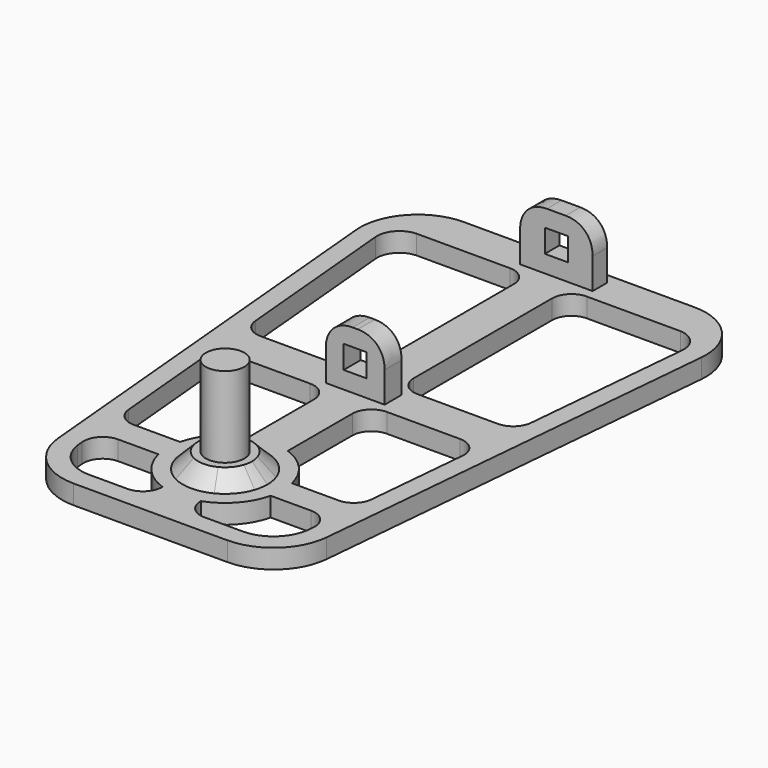
from build123d import *

# Parameters (mm, degrees)
F1_DEPTH    = 6.35
F2_DEPTH    = 25.4
F3_T1_DEPTH = 51.4821597159
F3_T3_DEPTH = 50.4775569558
F5_DEPTH    = 92.5147765378
F0_R        = 6.35
F6_DEPTH    = 11.43
F7_SIZE     = 5.07999
F8_DEPTH    = 38.1


# Not quite as in the source:
# - a fillet or chamfer that OpenCascade refuses, or shapes differently, is made with other operations: its cross-section is extruded or revolved along the edge and cut away or added
# - a fillet or chamfer is up to 0.001 mm smaller than in the source, because OpenCascade refuses the exact size


with BuildPart() as f1:
    # F0 (on Top) → F1 (new body)
    with BuildSketch(Plane.XY):
        with BuildLine():
            Line((38.1, 88.9586370111), (0, 88.9586370111))
            Line((0, 88.9586370111), (-38.1, 88.9586370111))
            ThreePointArc((-38.1, 88.9586370111), (-52.1700244652, 82.7514136403), (-57.0709376771, 68.1748481972))
            Line((-57.0709376771, 68.1748481972), (-44.3709376771, -70.7872367892))
            ThreePointArc((-44.3709376771, -70.7872367892), (-38.2427766292, -83.1234724406), (-25.4, -88.1034479753))
            Line((-25.4, -88.1034479753), (0, -88.1034479753))
            Line((0, -88.1034479753), (25.4, -88.1034479753))
            ThreePointArc((25.4, -88.1034479753), (38.2427766292, -83.1234724406), (44.3709376771, -70.7872367892))
            Line((44.3709376771, -70.7872367892), (57.0709376771, 68.1748481972))
            ThreePointArc((57.0709376771, 68.1748481972), (52.1700244652, 82.7514136403), (38.1, 88.9586370111))
        make_face()
        with BuildLine():
            Line((-12.7, -81.7534479753), (-25.4, -81.7534479753))
            ThreePointArc((-25.4, -81.7534479753), (-33.7498286884, -78.6277029444), (-37.9944737374, -70.7872367892))
            Line((-37.9944737374, -70.7872367892), (-38.1945348322, -68.5981890052))
            ThreePointArc((-38.1945348322, -68.5981890052), (-36.5608970949, -63.7393338575), (-31.8708889399, -61.6702594006))
            Line((-31.8708889399, -61.6702594006), (-18.54215425, -61.6702594006))
            ThreePointArc((-18.54215425, -61.6702594006), (-19.0498410445, -57.2231112436), (-18.5058372648, -52.7802594006))
            Line((-18.5058372648, -52.7802594006), (-33.8440386665, -52.7802594006))
            ThreePointArc((-33.8440386665, -52.7802594006), (-38.1249642095, -51.1202675557), (-40.1676845588, -47.0081890052))
            Line((-40.1676845588, -47.0081890052), (-43.2503548745, -13.2779296046))
            ThreePointArc((-43.2503548745, -13.2779296046), (-41.6167171372, -8.4190744569), (-36.9267089821, -6.35))
            Line((-36.9267089821, -6.35), (-12.7, -6.35))
            ThreePointArc((-12.7, -6.35), (-8.2098719395, -8.2098719395), (-6.35, -12.7))
            Line((-6.35, -12.7), (-6.35, -39.3404204633))
            ThreePointArc((-6.35, -39.3404204633), (0, -38.2509327054), (6.35, -39.3404204633))
            Line((6.35, -39.3404204633), (6.35, -12.7))
            ThreePointArc((6.35, -12.7), (8.2098719395, -8.2098719395), (12.7, -6.35))
            Line((12.7, -6.35), (36.9267089821, -6.35))
            ThreePointArc((36.9267089821, -6.35), (41.6167171372, -8.4190744569), (43.2503548745, -13.2779296046))
            Line((43.2503548745, -13.2779296046), (40.1676845588, -47.0081890052))
            ThreePointArc((40.1676845588, -47.0081890052), (38.1249642095, -51.1202675557), (33.8440386665, -52.7802594006))
            Line((33.8440386665, -52.7802594006), (18.5058372648, -52.7802594006))
            ThreePointArc((18.5058372648, -52.7802594006), (18.9134700663, -55.0242794484), (19.05, -57.3009327054))
            ThreePointArc((19.05, -57.3009327054), (18.9226126428, -59.5003032446), (18.54215425, -61.6702594006))
            Line((18.54215425, -61.6702594006), (31.8708889399, -61.6702594006))
            ThreePointArc((31.8708889399, -61.6702594006), (36.5608970949, -63.7393338575), (38.1945348322, -68.5981890052))
            Line((38.1945348322, -68.5981890052), (37.9944737374, -70.7872367892))
            ThreePointArc((37.9944737374, -70.7872367892), (33.7498286884, -78.6277029444), (25.4, -81.7534479753))
            Line((25.4, -81.7534479753), (12.7, -81.7534479753))
            ThreePointArc((12.7, -81.7534479753), (8.2098719395, -79.8935760359), (6.35, -75.4034479753))
            Line((6.35, -75.4034479753), (6.35, -75.2614449475))
            ThreePointArc((6.35, -75.2614449475), (0, -76.3509327054), (-6.35, -75.2614449475))
            Line((-6.35, -75.2614449475), (-6.35, -75.4034479753))
            ThreePointArc((-6.35, -75.4034479753), (-8.2098719395, -79.8935760359), (-12.7, -81.7534479753))
        make_face(mode=Mode.SUBTRACT)
        Polygon((-9.7281606868, 3.4770201892), (0, 3.4770201892), (9.7281606868, 3.4770201892), (9.7281606868, -3.5551395267), (0, -3.5551395267), (-9.7281606868, -3.5551395267), align=None, mode=Mode.SUBTRACT)
        with BuildLine():
            Line((-45.571707494, 12.1220703954), (-50.6944737374, 68.1748481972))
            ThreePointArc((-50.6944737374, 68.1748481972), (-48.902422759, 73.7198976746), (-43.6570607126, 76.2586370111))
            Line((-43.6570607126, 76.2586370111), (-12.7, 76.2586370111))
            ThreePointArc((-12.7, 76.2586370111), (-8.2098719395, 74.3987650716), (-6.35, 69.9086370111))
            Line((-6.35, 69.9086370111), (-6.35, 12.7))
            ThreePointArc((-6.35, 12.7), (-8.2098719395, 8.2098719395), (-12.7, 6.35))
            Line((-12.7, 6.35), (-39.2480616016, 6.35))
            ThreePointArc((-39.2480616016, 6.35), (-43.5289871447, 8.0099918449), (-45.571707494, 12.1220703954))
        make_face(mode=Mode.SUBTRACT)
        with BuildLine():
            Line((6.35, 12.7), (6.35, 69.9086370111))
            ThreePointArc((6.35, 69.9086370111), (8.2098719395, 74.3987650716), (12.7, 76.2586370111))
            Line((12.7, 76.2586370111), (43.6570607126, 76.2586370111))
            ThreePointArc((43.6570607126, 76.2586370111), (48.902422759, 73.7198976746), (50.6944737374, 68.1748481972))
            Line((50.6944737374, 68.1748481972), (45.571707494, 12.1220703954))
            ThreePointArc((45.571707494, 12.1220703954), (43.5289871447, 8.0099918449), (39.2480616016, 6.35))
            Line((39.2480616016, 6.35), (12.7, 6.35))
            ThreePointArc((12.7, 6.35), (8.2098719395, 8.2098719395), (6.35, 12.7))
        make_face(mode=Mode.SUBTRACT)
        Polygon((-11.9884992018, 85.6025964022), (0, 85.6025964022), (11.9884992018, 85.6025964022), (11.9884992018, 79.5750394464), (0, 79.5750394464), (-11.9884992018, 79.5750394464), align=None, mode=Mode.SUBTRACT)
        with BuildLine():
            Line((-6.35, -69.7443405987), (-6.35, -75.2614449475))
            ThreePointArc((-6.35, -75.2614449475), (0, -76.3509327054), (6.35, -75.2614449475))
            Line((6.35, -75.2614449475), (6.35, -69.7443405987))
            ThreePointArc((6.35, -69.7443405987), (0, -71.2709327054), (-6.35, -69.7443405987))
        make_face()
        with BuildLine():
            Line((6.35, -69.7443405987), (6.35, -75.2614449475))
            ThreePointArc((6.35, -75.2614449475), (14.1804413522, -70.021686734), (18.54215425, -61.6702594006))
            Line((18.54215425, -61.6702594006), (13.2691327611, -61.6702594006))
            ThreePointArc((13.2691327611, -61.6702594006), (10.6077938033, -66.3913458218), (6.35, -69.7443405987))
        make_face()
        with BuildLine():
            Line((13.2691327611, -61.6702594006), (18.54215425, -61.6702594006))
            ThreePointArc((18.54215425, -61.6702594006), (18.9226126428, -59.5003032446), (19.05, -57.3009327054))
            ThreePointArc((19.05, -57.3009327054), (18.9134700663, -55.0242794484), (18.5058372648, -52.7802594006))
            Line((18.5058372648, -52.7802594006), (13.2183362369, -52.7802594006))
            ThreePointArc((13.2183362369, -52.7802594006), (13.7808029017, -55.0095638164), (13.97, -57.3009327054))
            ThreePointArc((13.97, -57.3009327054), (13.7936703722, -59.5135234186), (13.2691327611, -61.6702594006))
        make_face()
        with BuildLine():
            ThreePointArc((18.5058372648, -52.7802594006), (14.1283572718, -44.522356071), (6.35, -39.3404204633))
            Line((6.35, -39.3404204633), (6.35, -44.8575248121))
            ThreePointArc((6.35, -44.8575248121), (10.555679827, -48.1500571522), (13.2183362369, -52.7802594006))
            Line((13.2183362369, -52.7802594006), (18.5058372648, -52.7802594006))
        make_face()
        with BuildLine():
            ThreePointArc((-6.35, -39.3404204633), (-14.1283572718, -44.522356071), (-18.5058372648, -52.7802594006))
            Line((-18.5058372648, -52.7802594006), (-13.2183362369, -52.7802594006))
            ThreePointArc((-13.2183362369, -52.7802594006), (-10.555679827, -48.1500571522), (-6.35, -44.8575248121))
            Line((-6.35, -44.8575248121), (-6.35, -39.3404204633))
        make_face()
        with BuildLine():
            ThreePointArc((-18.54215425, -61.6702594006), (-14.1804413522, -70.021686734), (-6.35, -75.2614449475))
            Line((-6.35, -75.2614449475), (-6.35, -69.7443405987))
            ThreePointArc((-6.35, -69.7443405987), (-10.6077938033, -66.3913458218), (-13.2691327611, -61.6702594006))
            Line((-13.2691327611, -61.6702594006), (-18.54215425, -61.6702594006))
        make_face()
        with BuildLine():
            ThreePointArc((-18.5058372648, -52.7802594006), (-19.0498410445, -57.2231112436), (-18.54215425, -61.6702594006))
            Line((-18.54215425, -61.6702594006), (-13.2691327611, -61.6702594006))
            ThreePointArc((-13.2691327611, -61.6702594006), (-13.9697719552, -57.221110899), (-13.2183362369, -52.7802594006))
            Line((-13.2183362369, -52.7802594006), (-18.5058372648, -52.7802594006))
        make_face()
        with BuildLine():
            ThreePointArc((6.35, -39.3404204633), (0, -38.2509327054), (-6.35, -39.3404204633))
            Line((-6.35, -39.3404204633), (-6.35, -44.8575248121))
            ThreePointArc((-6.35, -44.8575248121), (0, -43.3309327054), (6.35, -44.8575248121))
            Line((6.35, -44.8575248121), (6.35, -39.3404204633))
        make_face()
    extrude(amount=F1_DEPTH)

    # F0 (on Top) → F2 (join)
    with BuildSketch(Plane.XY):
        Polygon((9.7281606868, 3.4770201892), (0, 3.4770201892), (-9.7281606868, 3.4770201892), (-9.7281606868, -3.5551395267), (0, -3.5551395267), (9.7281606868, -3.5551395267), align=None)
        Polygon((11.9884992018, 85.6025964022), (0, 85.6025964022), (-11.9884992018, 85.6025964022), (-11.9884992018, 79.5750394464), (0, 79.5750394464), (11.9884992018, 79.5750394464), align=None)
    extrude(amount=F2_DEPTH)

    # F3: fillet of radius 8.89 on 4 edges, made by hand

    # F3_s2 → F3_t1 (cut)
    with BuildSketch(Plane.XZ.offset(-25.7020201892)):
        with BuildLine():
            add(Edge.make_bspline(
                [(-9.7281606868, 16.51), (-9.7281606868, 25.4), (-0.8381606868, 25.4)],
                knots=[0, 0, 0, 1, 1, 1], degree=2, weights=[1, 0.8181818182, 1]))
            Line((-0.8381606868, 25.4), (-9.7281606868, 25.4))
            Line((-9.7281606868, 25.4), (-9.7281606868, 16.51))
        make_face()
        with BuildLine():
            add(Edge.make_bspline(
                [(9.7281606868, 16.51), (9.7281606868, 25.4), (0.8381606868, 25.4)],
                knots=[0, 0, 0, 1, 1, 1], degree=2, weights=[1, 0.8181818182, 1]))
            Line((0.8381606868, 25.4), (9.7281606868, 25.4))
            Line((9.7281606868, 25.4), (9.7281606868, 16.51))
        make_face()
    extrude(amount=F3_T1_DEPTH, mode=Mode.SUBTRACT)

    # F3_s4 → F3_t3 (cut)
    with BuildSketch(Plane.XZ.offset(-107.8275964022)):
        with BuildLine():
            add(Edge.make_bspline(
                [(11.9884992018, 16.51), (11.9884992018, 25.4), (3.0984992018, 25.4)],
                knots=[0, 0, 0, 1, 1, 1], degree=2, weights=[1, 0.8181818182, 1]))
            Line((3.0984992018, 25.4), (11.9884992018, 25.4))
            Line((11.9884992018, 25.4), (11.9884992018, 16.51))
        make_face()
        with BuildLine():
            add(Edge.make_bspline(
                [(-11.9884992018, 16.51), (-11.9884992018, 25.4), (-3.0984992018, 25.4)],
                knots=[0, 0, 0, 1, 1, 1], degree=2, weights=[1, 0.8181818182, 1]))
            Line((-3.0984992018, 25.4), (-11.9884992018, 25.4))
            Line((-11.9884992018, 25.4), (-11.9884992018, 16.51))
        make_face()
    extrude(amount=F3_T3_DEPTH, mode=Mode.SUBTRACT)

    # F4 (on face) → F5 (cut, through all)
    with BuildSketch(Plane.XZ.offset(3.5551395267)):
        Polygon((3.81, 19.685), (0, 19.685), (-3.81, 19.685), (-3.81, 15.875), (-3.81, 12.065), (0, 12.065), (3.81, 12.065), (3.81, 15.875), align=None)
    extrude(amount=-F5_DEPTH, mode=Mode.SUBTRACT)

    # F0 (on Top) → F6 (join)
    with BuildSketch(Plane.XY):
        with BuildLine():
            Line((-6.35, -61.6702594006), (-6.35, -69.7443405987))
            ThreePointArc((-6.35, -69.7443405987), (0, -71.2709327054), (6.35, -69.7443405987))
            Line((6.35, -69.7443405987), (6.35, -61.6702594006))
            Line((6.35, -61.6702594006), (13.2691327611, -61.6702594006))
            ThreePointArc((13.2691327611, -61.6702594006), (13.7936703722, -59.5135234186), (13.97, -57.3009327054))
            ThreePointArc((13.97, -57.3009327054), (13.7808029017, -55.0095638164), (13.2183362369, -52.7802594006))
            Line((13.2183362369, -52.7802594006), (6.35, -52.7802594006))
            Line((6.35, -52.7802594006), (6.35, -44.8575248121))
            ThreePointArc((6.35, -44.8575248121), (0, -43.3309327054), (-6.35, -44.8575248121))
            Line((-6.35, -44.8575248121), (-6.35, -52.7802594006))
            Line((-6.35, -52.7802594006), (-13.2183362369, -52.7802594006))
            ThreePointArc((-13.2183362369, -52.7802594006), (-13.9697719552, -57.221110899), (-13.2691327611, -61.6702594006))
            Line((-13.2691327611, -61.6702594006), (-6.35, -61.6702594006))
        make_face()
        with Locations((0, -57.3009327054)):
            Circle(F0_R, mode=Mode.SUBTRACT)
        with BuildLine():
            ThreePointArc((-6.35, -44.8575248121), (-10.555679827, -48.1500571522), (-13.2183362369, -52.7802594006))
            Line((-13.2183362369, -52.7802594006), (-6.35, -52.7802594006))
            Line((-6.35, -52.7802594006), (-6.35, -44.8575248121))
        make_face()
        with BuildLine():
            ThreePointArc((-13.2691327611, -61.6702594006), (-10.6077938033, -66.3913458218), (-6.35, -69.7443405987))
            Line((-6.35, -69.7443405987), (-6.35, -61.6702594006))
            Line((-6.35, -61.6702594006), (-13.2691327611, -61.6702594006))
        make_face()
        with BuildLine():
            ThreePointArc((13.2183362369, -52.7802594006), (10.555679827, -48.1500571522), (6.35, -44.8575248121))
            Line((6.35, -44.8575248121), (6.35, -52.7802594006))
            Line((6.35, -52.7802594006), (13.2183362369, -52.7802594006))
        make_face()
        with BuildLine():
            Line((6.35, -61.6702594006), (6.35, -69.7443405987))
            ThreePointArc((6.35, -69.7443405987), (10.6077938033, -66.3913458218), (13.2691327611, -61.6702594006))
            Line((13.2691327611, -61.6702594006), (6.35, -61.6702594006))
        make_face()
    extrude(amount=F6_DEPTH)

    # F7 (size 5.08 in the source; OpenCascade refuses exactly that, so slightly less here)
    f7_edges = [f1.edges().sort_by_distance(p)[0] for p in [
        (-6.35, -44.857525, 11.43),
    ]]
    chamfer(f7_edges, length=F7_SIZE)

    # F0 (on Top) → F8 (join)
    with BuildSketch(Plane.XY):
        with Locations((0, -57.3009327054)):
            Circle(F0_R)
    extrude(amount=F8_DEPTH)


solid = f1.part
